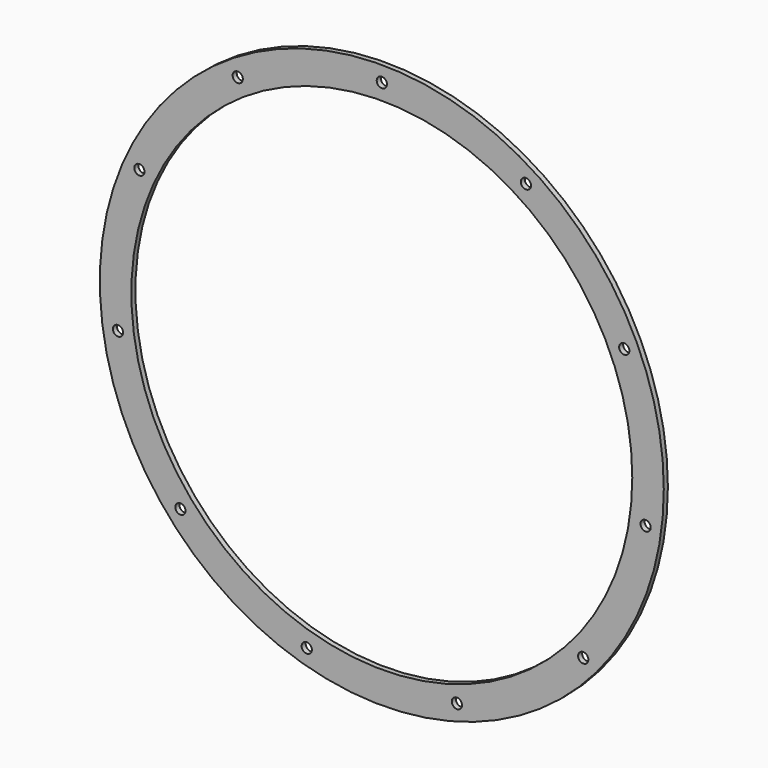
from build123d import *

# Parameters (mm, degrees)
F0_R            = 165.5
F0_R_2          = 147
F1_DEPTH        = 3
F2_R            = 3
F3_DEPTH        = 25
F3_COPIES_COUNT = 11


# Not quite as in the source:
# - a pattern or mirror of a feature is missing from the dataset's text; its kind, count and spacing are read off the source's solid


with BuildPart() as f1:
    # F0 (on Front) → F1 (new body)
    with BuildSketch(Plane.XZ):
        Circle(F0_R)
        Circle(F0_R_2, mode=Mode.SUBTRACT)
    extrude(amount=F1_DEPTH)

    # F2 (on face) → F3 (cut)
    with BuildSketch(Plane.XZ.offset(3)):
        with Locations((0, 156.4114242792)):
            Circle(F2_R)
    f3 = extrude(amount=-F3_DEPTH, mode=Mode.SUBTRACT)

    # F3_copies: F3 ×11 about axis
    f3_copies_axis = Axis((0, 0, 0), (0, 1, 0))
    for i in range(1, F3_COPIES_COUNT):
        add(f3.rotate(f3_copies_axis, i * 360 / F3_COPIES_COUNT), mode=Mode.SUBTRACT)


solid = f1.part
